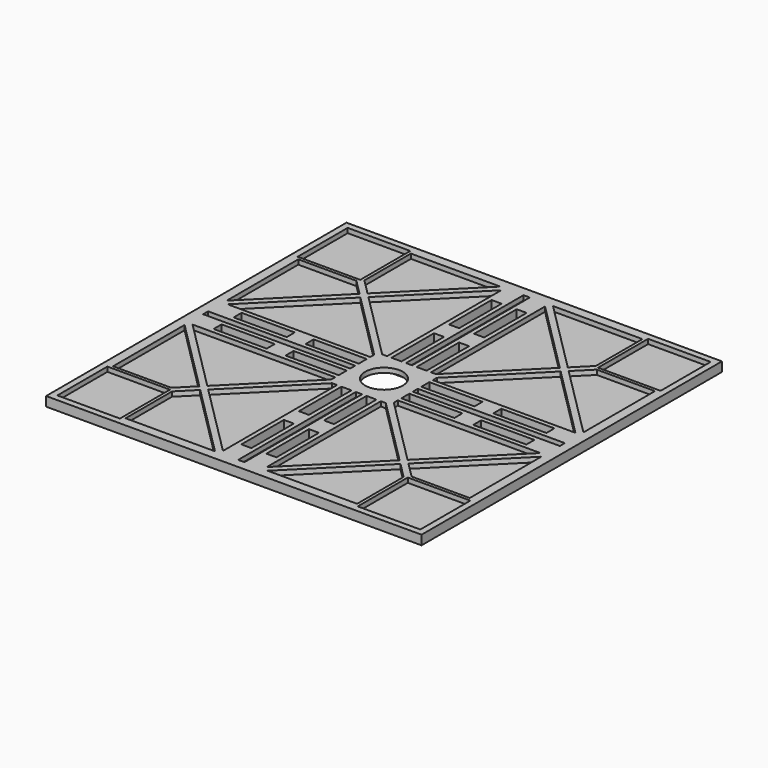
from build123d import *

# Parameters (mm, degrees)
F0_W             = 120
F0_H             = 120
F1_DEPTH         = 3
F2_W             = 114
F2_H             = 114
F3_DEPTH         = 1.5
F5_W             = 57.1697762102
F5_H             = 6
F6_DEPTH         = 1.5
F6_COPIES_COUNT  = 4
F8_W             = 16.9853664327
F8_H             = 3.2
F9_DEPTH         = 3
F9_COPIES_COUNT  = 4
F10_W            = 22
F10_H            = 22
F10_W_2          = 15
F10_H_2          = 15
F11_DEPTH        = 1.5
F11_COPIES_COUNT = 4
F12_W            = 20
F12_H            = 20
F12_W_2          = 14
F12_H_2          = 14
F13_DEPTH        = 1.5
F13_COPIES_COUNT = 4
F16_DEPTH        = 1.5
F16_COPIES_COUNT = 4
F18_DEPTH        = 1.5
F18_COPIES_COUNT = 4
F19_W            = 20
F19_H            = 20
F20_DEPTH        = 1.5
F21_R            = 6
F22_DEPTH        = 3
F23_W            = 16
F23_H            = 16
F24_DEPTH        = 1.5


# Not quite as in the source:
# - a pattern or mirror of a feature is missing from the dataset's text; its kind, count and spacing are read off the source's solid


with BuildPart() as f1:
    # F0 (on Top) → F1 (new body)
    with BuildSketch(Plane.XY):
        Rectangle(F0_W, F0_H)
    extrude(amount=F1_DEPTH)

    # F2 (on face) → F3 (cut)
    with BuildSketch(Plane.XY.offset(3)):
        Rectangle(F2_W, F2_H)
    extrude(amount=-F3_DEPTH, mode=Mode.SUBTRACT)

    # F5 (on face) → F6 (join)
    with BuildSketch(Plane.XY.offset(1.5)):
        with Locations((28.4151118949, -4)):
            Rectangle(F5_W, F5_H)
        with Locations((28.4151118949, 4)):
            Rectangle(F5_W, F5_H)
    f6 = extrude(amount=F6_DEPTH)

    # F6_copies: F6 ×4 about axis
    f6_copies_axis = Axis((0, 0, 0), (0, 0, 1))
    for i in range(1, F6_COPIES_COUNT):
        add(f6.rotate(f6_copies_axis, i * 360 / F6_COPIES_COUNT))

    # F8 (on face) → F9 (cut)
    with BuildSketch(Plane.XY.offset(3)):
        with Locations((18.4926832163, -4)):
            Rectangle(F8_W, F8_H)
        with Locations((41.4926832163, -4)):
            Rectangle(F8_W, F8_H)
        with Locations((41.4926832163, 4)):
            Rectangle(F8_W, F8_H)
        with Locations((18.4926832163, 4)):
            Rectangle(F8_W, F8_H)
    f9 = extrude(amount=-F9_DEPTH, mode=Mode.SUBTRACT)

    # F9_copies: F9 ×4 about axis
    f9_copies_axis = Axis((0, 0, 0), (0, 0, 1))
    for i in range(1, F9_COPIES_COUNT):
        add(f9.rotate(f9_copies_axis, i * 360 / F9_COPIES_COUNT), mode=Mode.SUBTRACT)

    # F10 (on face) → F11 (join)
    with BuildSketch(Plane.XY.offset(1.5)):
        with Locations((-48, 48)):
            Rectangle(F10_W, F10_H)
        with Locations((-48, 48)):
            Rectangle(F10_W_2, F10_H_2, mode=Mode.SUBTRACT)
    f11 = extrude(amount=F11_DEPTH)

    # F11_copies: F11 ×4 about axis
    f11_copies_axis = Axis((0, 0, 0), (0, 0, 1))
    for i in range(1, F11_COPIES_COUNT):
        add(f11.rotate(f11_copies_axis, i * 360 / F11_COPIES_COUNT))

    # F12 (on face) → F13 (cut)
    with BuildSketch(Plane.XY.offset(3)):
        with Locations((-48, 48)):
            Rectangle(F12_W, F12_H)
        with Locations((-48, 48)):
            Rectangle(F12_W_2, F12_H_2, mode=Mode.SUBTRACT)
    f13 = extrude(amount=-F13_DEPTH, mode=Mode.SUBTRACT)

    # F13_copies: F13 ×4 about axis
    f13_copies_axis = Axis((0, 0, 0), (0, 0, 1))
    for i in range(1, F13_COPIES_COUNT):
        add(f13.rotate(f13_copies_axis, i * 360 / F13_COPIES_COUNT), mode=Mode.SUBTRACT)

    # F15 (on face) → F16 (join)
    with BuildSketch(Plane.XY.offset(3)):
        Polygon((-7, 7), (-7, 8.4142135624), (-37, 38.4142135624), (-37, 37), (-38.4142135624, 37), (-8.4142135624, 7), align=None)
    f16 = extrude(amount=-F16_DEPTH)

    # F16_copies: F16 ×4 about axis
    f16_copies_axis = Axis((0, 0, 0), (0, 0, 1))
    for i in range(1, F16_COPIES_COUNT):
        add(f16.rotate(f16_copies_axis, i * 360 / F16_COPIES_COUNT))

    # F17 (on face) → F18 (join)
    with BuildSketch(Plane.XY.offset(3)):
        Polygon((-7, 55.5857864376), (-7, 57), (-8.4142135624, 57), (-57, 8.4142135624), (-57, 7), (-55.5857864376, 7), align=None)
    f18 = extrude(amount=-F18_DEPTH)

    # F18_copies: F18 ×4 about axis
    f18_copies_axis = Axis((0, 0, 0), (0, 0, 1))
    for i in range(1, F18_COPIES_COUNT):
        add(f18.rotate(f18_copies_axis, i * 360 / F18_COPIES_COUNT))

    # F19 (on face) → F20 (join)
    with BuildSketch(Plane.XY.offset(3)):
        Rectangle(F19_W, F19_H)
    extrude(amount=-F20_DEPTH)

    # F21 (on face) → F22 (cut)
    with BuildSketch(Plane(origin=(0, 0, 0), x_dir=(1, 0, 0), z_dir=(0, 0, -1))):
        Circle(F21_R)
    extrude(amount=-F22_DEPTH, mode=Mode.SUBTRACT)

    # F23 (on face) → F24 (cut)
    with BuildSketch(Plane(origin=(0, 0, 0), x_dir=(1, 0, 0), z_dir=(0, 0, -1))):
        Rectangle(F23_W, F23_H)
    extrude(amount=-F24_DEPTH, mode=Mode.SUBTRACT)


solid = f1.part
